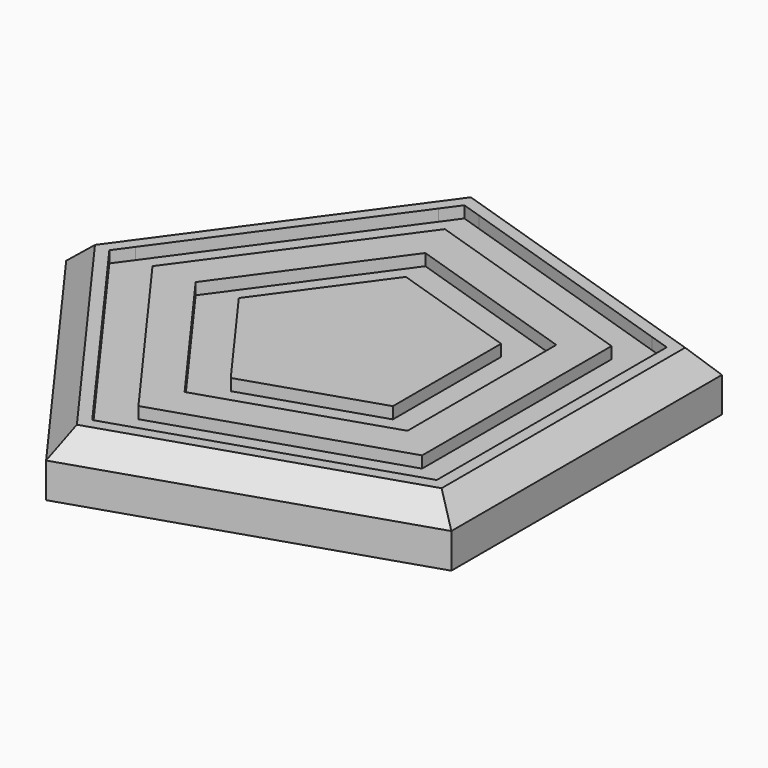
from build123d import *

# Parameters (mm, degrees)
F0_R     = 3.8339233168
F0_R_2   = 3.175
F1_DEPTH = 2.5
F2_SIZE  = 1
F3_DEPTH = 3
F4_DEPTH = 1.5
F5_DEPTH = 2


with BuildPart() as f1:
    # F0 (on Top) → F1 (new body)
    with BuildSketch(Plane.XY):
        Polygon((4, -2.906170112), (4, 2.906170112), (-1.527864045, 4.7022820183), (-4.94427191, 0), (-1.527864045, -4.7022820183), align=None)
        Circle(F0_R, mode=Mode.SUBTRACT)
        Circle(F0_R)
        Circle(F0_R_2, mode=Mode.SUBTRACT)
        Circle(F0_R_2)
    extrude(amount=F1_DEPTH)

    # F0 (on Top) → F3 (join)
    with BuildSketch(Plane.XY):
        Circle(F0_R_2)
    extrude(amount=-F3_DEPTH)

    # F0 (on Top) → F4 (join)
    with BuildSketch(Plane.XY):
        Circle(F0_R)
        Circle(F0_R_2, mode=Mode.SUBTRACT)
    extrude(amount=-F4_DEPTH)


with BuildPart() as f1b:
    # F0 (on Top) → F1, piece 2 (new body)
    with BuildSketch(Plane.XY):
        Polygon((7, -5.085797696), (7, 5.085797696), (-2.6737620788, 8.2289935321), (-8.6524758425, 0), (-2.6737620788, -8.2289935321), align=None)
        Polygon((-2.1008130619, 6.4656377752), (5.5, 3.995983904), (5.5, -3.995983904), (-2.1008130619, -6.4656377752), (-6.7983738762, 0), align=None, mode=Mode.SUBTRACT)
    extrude(amount=F1_DEPTH)


with BuildPart() as f1c:
    # F0 (on Top) → F1, piece 3 (new body)
    with BuildSketch(Plane.XY):
        with BuildLine():
            ThreePointArc((-8.0901700058, -5.8778524375), (-6.1711601329, -7.8687217904), (-3.7802935026, -9.2579361109))
            Line((-3.7802935026, -9.2579361109), (-9.9729954018, -0.734413178))
            ThreePointArc((-9.9729954018, -0.734413178), (-9.390592526, -3.4375532011), (-8.0901700058, -5.8778524375))
        make_face()
        with BuildLine():
            ThreePointArc((-9.9729954018, 0.734413178), (-9.3905925168, 3.4375532262), (-8.0901699744, 5.8778524807))
            Line((-8.0901699744, 5.8778524807), (-12.360679775, 0))
            Line((-12.360679775, 0), (-8.0901700058, -5.8778524375))
            ThreePointArc((-8.0901700058, -5.8778524375), (-9.390592526, -3.4375532011), (-9.9729954018, -0.734413178))
            Line((-9.9729954018, -0.734413178), (-10.5065778087, 0))
            Line((-10.5065778087, 0), (-9.9729954018, 0.734413178))
        make_face()
        with BuildLine():
            Line((-3.8196601125, -11.7557050458), (3.0901696906, -9.5105652452))
            ThreePointArc((3.0901696906, -9.5105652452), (0.367454614, -9.9932465749), (-2.3833566254, -9.7118284167))
            Line((-2.3833566254, -9.7118284167), (-3.2467110956, -9.992349289))
            Line((-3.2467110956, -9.992349289), (-3.7802935026, -9.2579361109))
            ThreePointArc((-3.7802935026, -9.2579361109), (-6.1711601329, -7.8687217904), (-8.0901700058, -5.8778524375))
            Line((-8.0901700058, -5.8778524375), (-3.8196601125, -11.7557050458))
        make_face()
        with BuildLine():
            ThreePointArc((3.0901696906, -9.5105652452), (5.5766057109, -8.3006908595), (7.6366455297, -6.4561323603))
            Line((7.6366455297, -6.4561323603), (-2.3833566254, -9.7118284167))
            ThreePointArc((-2.3833566254, -9.7118284167), (0.367454614, -9.9932465749), (3.0901696906, -9.5105652452))
        make_face()
        with BuildLine():
            Line((10, -7.2654252801), (10, 0))
            ThreePointArc((10, 0), (9.6176920308, -2.7386127875), (8.5, -5.2678268764))
            Line((8.5, -5.2678268764), (8.5, -6.175611488))
            Line((8.5, -6.175611488), (7.6366455297, -6.4561323603))
            ThreePointArc((7.6366455297, -6.4561323603), (5.5766057109, -8.3006908595), (3.0901696906, -9.5105652452))
            Line((3.0901696906, -9.5105652452), (10, -7.2654252801))
        make_face()
        with BuildLine():
            ThreePointArc((8.5, -5.2678268764), (9.6176920308, -2.7386127875), (10, 0))
            ThreePointArc((10, 0), (9.6176920308, 2.7386127875), (8.5, 5.2678268764))
            Line((8.5, 5.2678268764), (8.5, -5.2678268764))
        make_face()
        with BuildLine():
            ThreePointArc((8.5, 5.2678268764), (9.6176920308, 2.7386127875), (10, 0))
            Line((10, 0), (10, 7.2654252801))
            Line((10, 7.2654252801), (3.0901697709, 9.5105652191))
            ThreePointArc((3.0901697709, 9.5105652191), (5.5766057459, 8.300690836), (7.6366455297, 6.4561323603))
            Line((7.6366455297, 6.4561323603), (8.5, 6.175611488))
            Line((8.5, 6.175611488), (8.5, 5.2678268764))
        make_face()
        with BuildLine():
            ThreePointArc((-2.3833566254, 9.7118284167), (0.3674546562, 9.9932465733), (3.0901697709, 9.5105652191))
            Line((3.0901697709, 9.5105652191), (-3.8196601125, 11.7557050458))
            Line((-3.8196601125, 11.7557050458), (-8.0901699744, 5.8778524807))
            ThreePointArc((-8.0901699744, 5.8778524807), (-6.1711601119, 7.8687218068), (-3.7802935026, 9.2579361109))
            Line((-3.7802935026, 9.2579361109), (-3.2467110956, 9.992349289))
            Line((-3.2467110956, 9.992349289), (-2.3833566254, 9.7118284167))
        make_face()
        with BuildLine():
            Line((-9.9729954018, 0.734413178), (-3.7802935026, 9.2579361109))
            ThreePointArc((-3.7802935026, 9.2579361109), (-6.1711601119, 7.8687218068), (-8.0901699744, 5.8778524807))
            ThreePointArc((-8.0901699744, 5.8778524807), (-9.3905925168, 3.4375532262), (-9.9729954018, 0.734413178))
        make_face()
        with BuildLine():
            Line((-2.3833566254, 9.7118284167), (7.6366455297, 6.4561323603))
            ThreePointArc((7.6366455297, 6.4561323603), (5.5766057459, 8.300690836), (3.0901697709, 9.5105652191))
            ThreePointArc((3.0901697709, 9.5105652191), (0.3674546562, 9.9932465733), (-2.3833566254, 9.7118284167))
        make_face()
    extrude(amount=F1_DEPTH)

    # F2
    f2_edges = [f1c.edges().sort_by_distance(p)[0] for p in [
        (3.09017, 9.510565, 2.5),
        (-8.09017, 5.877853, 2.5),
        (-8.09017, -5.877853, 2.5),
        (3.09017, -9.510565, 2.5),
        (10, 0, 2.5),
    ]]
    chamfer(f2_edges, length=F2_SIZE)


with BuildPart() as f5:
    # F0 (on Top) → F5 (new body)
    with BuildSketch(Plane.XY):
        with BuildLine():
            Line((8.5, -5.2678268764), (8.5, 5.2678268764))
            ThreePointArc((8.5, 5.2678268764), (8.0901699437, 5.8778525229), (7.6366455297, 6.4561323603))
            Line((7.6366455297, 6.4561323603), (-2.3833566254, 9.7118284167))
            ThreePointArc((-2.3833566254, 9.7118284167), (-3.0901699437, 9.510565163), (-3.7802935026, 9.2579361109))
            Line((-3.7802935026, 9.2579361109), (-9.9729954018, 0.734413178))
            ThreePointArc((-9.9729954018, 0.734413178), (-10, 0), (-9.9729954018, -0.734413178))
            Line((-9.9729954018, -0.734413178), (-3.7802935026, -9.2579361109))
            ThreePointArc((-3.7802935026, -9.2579361109), (-3.0901699437, -9.510565163), (-2.3833566254, -9.7118284167))
            Line((-2.3833566254, -9.7118284167), (7.6366455297, -6.4561323603))
            ThreePointArc((7.6366455297, -6.4561323603), (8.0901699437, -5.8778525229), (8.5, -5.2678268764))
        make_face()
        Polygon((-2.6737620788, 8.2289935321), (7, 5.085797696), (7, -5.085797696), (-2.6737620788, -8.2289935321), (-8.6524758425, 0), align=None, mode=Mode.SUBTRACT)
        with BuildLine():
            ThreePointArc((-9.9729954018, -0.734413178), (-10, 0), (-9.9729954018, 0.734413178))
            Line((-9.9729954018, 0.734413178), (-10.5065778087, 0))
            Line((-10.5065778087, 0), (-9.9729954018, -0.734413178))
        make_face()
        with BuildLine():
            ThreePointArc((-3.7802935026, 9.2579361109), (-3.0901699437, 9.510565163), (-2.3833566254, 9.7118284167))
            Line((-2.3833566254, 9.7118284167), (-3.2467110956, 9.992349289))
            Line((-3.2467110956, 9.992349289), (-3.7802935026, 9.2579361109))
        make_face()
        with BuildLine():
            ThreePointArc((7.6366455297, 6.4561323603), (8.0901699437, 5.8778525229), (8.5, 5.2678268764))
            Line((8.5, 5.2678268764), (8.5, 6.175611488))
            Line((8.5, 6.175611488), (7.6366455297, 6.4561323603))
        make_face()
        with BuildLine():
            Line((8.5, -6.175611488), (8.5, -5.2678268764))
            ThreePointArc((8.5, -5.2678268764), (8.0901699437, -5.8778525229), (7.6366455297, -6.4561323603))
            Line((7.6366455297, -6.4561323603), (8.5, -6.175611488))
        make_face()
        with BuildLine():
            Line((-3.2467110956, -9.992349289), (-2.3833566254, -9.7118284167))
            ThreePointArc((-2.3833566254, -9.7118284167), (-3.0901699437, -9.510565163), (-3.7802935026, -9.2579361109))
            Line((-3.7802935026, -9.2579361109), (-3.2467110956, -9.992349289))
        make_face()
    extrude(amount=F5_DEPTH)


with BuildPart() as f5b:
    # F0 (on Top) → F5, piece 2 (new body)
    with BuildSketch(Plane.XY):
        Polygon((5.5, -3.995983904), (5.5, 3.995983904), (-2.1008130619, 6.4656377752), (-6.7983738762, 0), (-2.1008130619, -6.4656377752), align=None)
        Polygon((-1.527864045, 4.7022820183), (4, 2.906170112), (4, -2.906170112), (-1.527864045, -4.7022820183), (-4.94427191, 0), align=None, mode=Mode.SUBTRACT)
    extrude(amount=F5_DEPTH)


solid = Compound([f1.part, f1b.part, f1c.part, f5.part, f5b.part])
